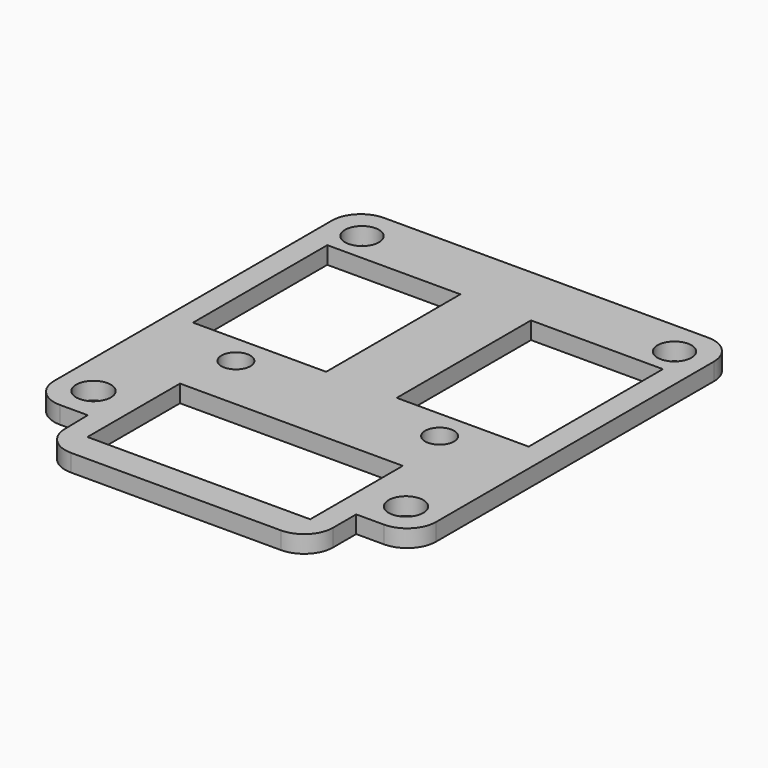
from build123d import *

# Parameters (mm, degrees)
F0_R     = 3
F0_R_2   = 2.5
F0_W     = 38.5
F0_H     = 20
F0_W_2   = 23
F0_H_2   = 29
F0_R_3   = 2.9306388833
F0_W_3   = 22.8
F1_DEPTH = 3


# Not quite as in the source:
# - a feature names something its author has since deleted; it is built from what else it names


with BuildPart() as f1:
    # F0 (on Top) → F1 (new body)
    with BuildSketch(Plane.XY):
        with BuildLine():
            ThreePointArc((-0.0987510204, 4.899238456), (1.4005055782, 1.429019202), (4.9002335876, 0))
            Line((4.9002335876, 0), (41.2, 0))
            ThreePointArc((41.2, 0), (44.7355339059, 1.4644660941), (46.2, 5))
            Line((46.2, 5), (46.2, 10))
            Line((46.2, 10), (51, 10))
            ThreePointArc((51, 10), (54.5355339059, 11.4644660941), (56, 15))
            Line((56, 15), (56, 30))
            Line((56, 30), (56, 75))
            ThreePointArc((56, 75), (54.5355339059, 78.5355339059), (51, 80))
            Line((51, 80), (-5, 80))
            ThreePointArc((-5, 80), (-8.5355339059, 78.5355339059), (-10, 75))
            Line((-10, 75), (-10, 30))
            Line((-10, 30), (-10, 15))
            ThreePointArc((-10, 15), (-8.5355339059, 11.4644660941), (-5, 10))
            Line((-5, 10), (-0.2015640213, 10))
            Line((-0.2015640213, 10), (-0.0987510204, 4.899238456))
        make_face()
        with Locations((-4, 16)):
            Circle(F0_R, mode=Mode.SUBTRACT)
        with Locations((5.5, 34.8868072033)):
            Circle(F0_R_2, mode=Mode.SUBTRACT)
        with Locations((23, 15)):
            Rectangle(F0_W, F0_H, mode=Mode.SUBTRACT)
        with Locations((50, 16)):
            Circle(F0_R, mode=Mode.SUBTRACT)
        with Locations((40.7, 34.8868072033)):
            Circle(F0_R_2, mode=Mode.SUBTRACT)
        with Locations((5.5, 54.5)):
            Rectangle(F0_W_2, F0_H_2, mode=Mode.SUBTRACT)
        with Locations((-4, 74)):
            Circle(F0_R_3, mode=Mode.SUBTRACT)
        with Locations((40.6, 54.5)):
            Rectangle(F0_W_3, F0_H_2, mode=Mode.SUBTRACT)
        with Locations((50, 74)):
            Circle(F0_R_3, mode=Mode.SUBTRACT)
    extrude(amount=F1_DEPTH)


solid = f1.part
